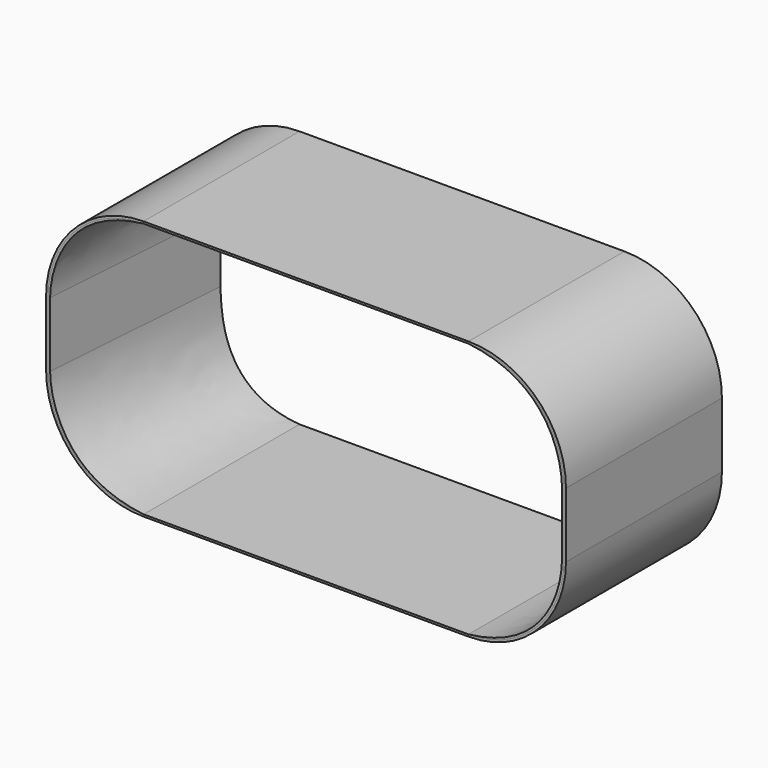
from build123d import *

# Parameters (mm, degrees)
F1_DEPTH = 152.4
F7_DEPTH = 1.5875
F9_DEPTH = 1.6002


# Not quite as in the source:
# - ends of sketch curves that miss each other by under 0.0002 mm in the source are joined


with BuildPart() as f1:
    # F0 (on Front) → F1 (new body)
    with BuildSketch(Plane.XZ):
        with BuildLine():
            Line((-127, -101.6), (127, -101.6))
            ThreePointArc((127, -101.6), (180.8815367264, -79.2815367264), (203.2, -25.4))
            Line((203.2, -25.4), (203.2, 25.4))
            ThreePointArc((203.2, 25.4), (180.8815367264, 79.2815367264), (127, 101.6))
            Line((127, 101.6), (-127, 101.6))
            ThreePointArc((-127, 101.6), (-180.8815367264, 79.2815367264), (-203.2, 25.4))
            Line((-203.2, 25.4), (-203.2, -25.4))
            ThreePointArc((-203.2, -25.4), (-180.8815367264, -79.2815367264), (-127, -101.6))
        make_face()
        with BuildLine():
            ThreePointArc((127, 100.0160425901), (179.7615097008, 78.1615097008), (201.6160425901, 25.4))
            Line((201.6160425901, 25.4), (201.6160425901, -25.4))
            ThreePointArc((201.6160425901, -25.4), (179.7615097008, -78.1615097008), (127, -100.0160425901))
            Line((127, -100.0160425901), (-127, -100.0160425901))
            ThreePointArc((-127, -100.0160425901), (-179.7615097008, -78.1615097008), (-201.6160425901, -25.4))
            Line((-201.6160425901, -25.4), (-201.6160425901, 25.4))
            ThreePointArc((-201.6160425901, 25.4), (-179.7615097008, 78.1615097008), (-127, 100.0160425901))
            Line((-127, 100.0160425901), (127, 100.0160425901))
        make_face(mode=Mode.SUBTRACT)
    extrude(amount=F1_DEPTH)


with BuildPart() as f4:
    # F2 (on face) → F4 section 0
    with BuildSketch(Plane.XZ.offset(152.4)):
        with BuildLine():
            add(Edge.make_bspline(
                [(-200.0462481144, 25.3999990709), (-200.1293383282, 40.9304278155), (-191.8294578791, 92.6911234856), (-127, 100.0160425901)],
                knots=[0, 0, 0, 0, 104.4189078379, 104.4189078379, 104.4189078379, 104.4189078379], degree=3))
            ThreePointArc((-127, 100.0160425901), (-179.7615097008, 78.1615097008), (-201.6160425901, 25.4))
            Line((-201.6160425901, 25.4), (-201.6160425901, -25.4))
            ThreePointArc((-201.6160425901, -25.4), (-179.7615097008, -78.1615097008), (-127, -100.0160425901))
            add(Edge.make_bspline(
                [(-200.0462481144, -25.3999990709), (-200.1293383282, -40.9304278155), (-191.8294578791, -92.6911234856), (-127, -100.0160425901)],
                knots=[0, 0, 0, 0, 104.4189078379, 104.4189078379, 104.4189078379, 104.4189078379], degree=3))
            Line((-200.0462481144, -25.3999990709), (-200.0462481144, 25.3999990709))
        make_face()
    # F3 (on face) → F4 section 1
    with BuildSketch(Plane(origin=(0, 0, 0), x_dir=(-1, 0, 0), z_dir=(0, 1, 0))):
        with BuildLine():
            Line((188.9160425901, 25.4), (188.9160425901, -25.4))
            add(Edge.make_bspline(
                [(188.9160425901, -25.4), (187.5226431005, -38.4616232589), (190.9089535475, -94.981238246), (127, -100.0160425901)],
                knots=[0, 0, 0, 0, 96.9595283705, 96.9595283705, 96.9595283705, 96.9595283705], degree=3))
            add(Edge.make_bspline(
                [(190.4939562082, -25.4), (189.0110522509, -35.2551564574), (193.8259601593, -96.4445024729), (127, -100.0160425901)],
                knots=[0, 0, 0, 0, 97.9746716595, 97.9746716595, 97.9746716595, 97.9746716595], degree=3))
            Line((190.4939562082, -25.4), (190.4939562082, 25.4))
            add(Edge.make_bspline(
                [(190.4939562082, 25.4), (189.0110522509, 35.2551564574), (193.8259601593, 96.4445024729), (127, 100.0160425901)],
                knots=[0, 0, 0, 0, 97.9746716595, 97.9746716595, 97.9746716595, 97.9746716595], degree=3))
            add(Edge.make_bspline(
                [(188.9160425901, 25.4), (187.5226431005, 38.4616232589), (190.9089535475, 94.981238246), (127, 100.0160425901)],
                knots=[0, 0, 0, 0, 96.9595283705, 96.9595283705, 96.9595283705, 96.9595283705], degree=3))
        make_face()
    loft()


with BuildPart() as f7:
    # F6 (on face) → F7 (new body)
    with BuildSketch(Plane(origin=(0, 0, 0), x_dir=(-1, 0, 0), z_dir=(0, 1, 0))):
        with BuildLine():
            Line((190.4939562082, 25.4), (190.4939562082, -25.4))
            add(Edge.make_bspline(
                [(201.6160425901, -25.4), (197.9086804628, -25.4), (194.2013183355, -25.4), (190.4939562082, -25.4)],
                knots=[0, 0, 0, 0, 1, 1, 1, 1], degree=3))
            Line((201.6160425901, -25.4), (201.6160425901, 25.4))
            add(Edge.make_bspline(
                [(201.6160425901, 25.4), (197.9086804628, 25.4), (194.2013183355, 25.4), (190.4939562082, 25.4)],
                knots=[0, 0, 0, 0, 1, 1, 1, 1], degree=3))
        make_face()
    extrude(amount=-F7_DEPTH)

    # F8 (on face) → F9 (cut)
    with BuildSketch(Plane(origin=(0, 0, 0), x_dir=(-1, 0, 0), z_dir=(0, 1, 0))):
        with BuildLine():
            Line((194.8643743992, 7.540625), (194.8643743992, 3.7859462056))
            ThreePointArc((194.8643743992, 3.7859462056), (196.0549993992, -3.96875), (197.2456243992, 3.7859462056))
            Line((197.2456243992, 3.7859462056), (197.2456243992, 7.540625))
            ThreePointArc((197.2456243992, 7.540625), (196.0549993992, 8.73125), (194.8643743992, 7.540625))
        make_face()
    extrude(amount=-F9_DEPTH, mode=Mode.SUBTRACT)


with BuildPart() as f10_1:
    # F10: instance of F7
    add(f7.part.mirror(Plane.YZ))


with BuildPart() as f10_2:
    # F10: instance of F4
    add(f4.part.mirror(Plane.YZ))


solid = Compound([f1.part, f4.part, f7.part, f10_1.part, f10_2.part])
